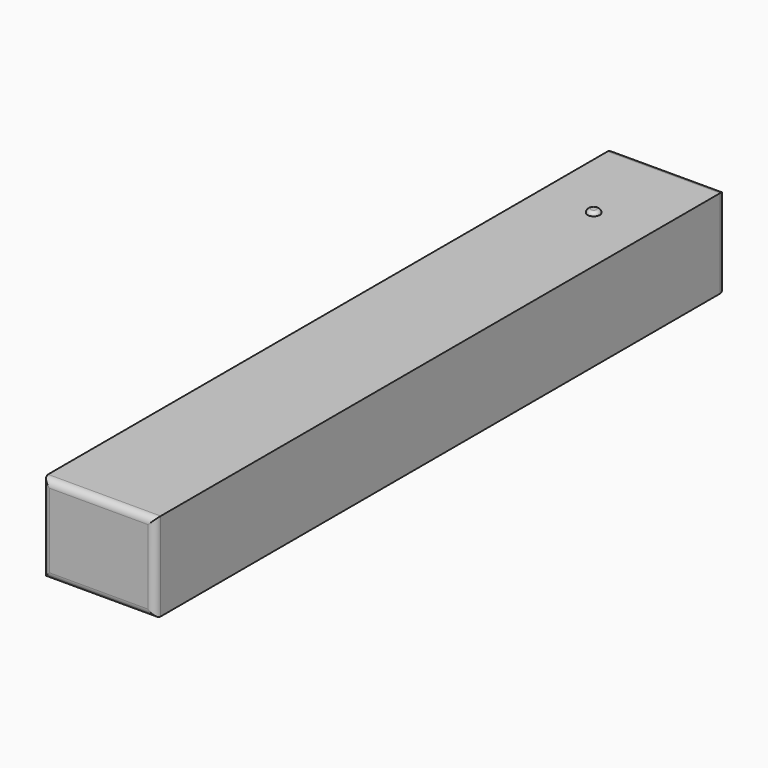
from build123d import *

# Parameters (mm, degrees)
F0_W      = 32.1
F0_H      = 25.2
F0_W_2    = 5.4
F0_H_2    = 5.4
F1_DEPTH  = 200
F3_W      = 32.1
F3_H      = 25.2
F4_DEPTH  = 3
F5_R      = 2
F6_R      = 1.75
F7_R      = 1.75
F8_DEPTH  = 1
F9_R      = 0.99999
F10_R     = 1.75
F11_DEPTH = 1
F12_R     = 0.99999


# Not quite as in the source:
# - a fillet or chamfer is up to 0.001 mm smaller than in the source, because OpenCascade refuses the exact size


with BuildPart() as f1:
    # F0 (on Front) → F1 (new body)
    with BuildSketch(Plane.XZ):
        with Locations((-0.710526225, -0.3999928176)):
            Rectangle(F0_W, F0_H)
        Polygon((-13.760526225, -6.9499006331), (-13.760526225, -4.5999928176), (-8.360526225, -4.5999928176), (-8.360526225, -9.9999928176), (-13.760526225, -9.9999928176), align=None, mode=Mode.SUBTRACT)
        with Locations((-4.160526225, -7.2999928176)):
            Rectangle(F0_W_2, F0_H_2, mode=Mode.SUBTRACT)
        Polygon((-13.760526225, -3.0999928176), (-13.760526225, 0.7499149978), (-13.760526225, 2.3000071824), (-8.360526225, 2.3000071824), (-8.360526225, -3.0999928176), align=None, mode=Mode.SUBTRACT)
        with Locations((-4.160526225, -0.3999928176)):
            Rectangle(F0_W_2, F0_H_2, mode=Mode.SUBTRACT)
        with Locations((2.739473775, -7.2999928176)):
            Rectangle(F0_W_2, F0_H_2, mode=Mode.SUBTRACT)
        with Locations((9.639473775, -7.2999928176)):
            Rectangle(F0_W_2, F0_H_2, mode=Mode.SUBTRACT)
        with Locations((2.739473775, -0.3999928176)):
            Rectangle(F0_W_2, F0_H_2, mode=Mode.SUBTRACT)
        with Locations((9.639473775, -0.3999928176)):
            Rectangle(F0_W_2, F0_H_2, mode=Mode.SUBTRACT)
        with Locations((-11.060526225, 6.5000071824)):
            Rectangle(F0_W_2, F0_H_2, mode=Mode.SUBTRACT)
        with Locations((-4.160526225, 6.5000071824)):
            Rectangle(F0_W_2, F0_H_2, mode=Mode.SUBTRACT)
        with Locations((2.739473775, 6.5000071824)):
            Rectangle(F0_W_2, F0_H_2, mode=Mode.SUBTRACT)
        with Locations((9.639473775, 6.5000071824)):
            Rectangle(F0_W_2, F0_H_2, mode=Mode.SUBTRACT)
    extrude(amount=F1_DEPTH)

    # F3 (on face) → F4 (join)
    with BuildSketch(Plane.XZ.offset(200)):
        with Locations((-0.710526225, -0.3999928176)):
            Rectangle(F3_W, F3_H)
    extrude(amount=F4_DEPTH)

    # F5
    f5_edges = [f1.edges().sort_by_distance(p)[0] for p in [
        (15.339474, -203, -0.399993),
        (-0.710526, -203, 12.200007),
        (-16.760526, -203, -0.399993),
        (-0.710526, -203, -12.999993),
    ]]
    fillet(f5_edges, radius=F5_R)

    # F6
    f6_edges = [f1.edges().sort_by_distance(p)[0] for p in [
        (-0.710526, 0, 12.200007),
        (15.339474, 0, -0.399993),
        (-0.710526, 0, -12.999993),
        (-16.760526, 0, -0.399993),
    ]]
    fillet(f6_edges, radius=F6_R)

    # F7 (on face) → F8 (join)
    with BuildSketch(Plane.XY.offset(12.2000071824)):
        with Locations((-0.710526225, -26.75)):
            Circle(F7_R)
    extrude(amount=F8_DEPTH)

    # F9 (radius 1 in the source; OpenCascade refuses exactly that, so slightly less here)
    f9_edges = [f1.edges().sort_by_distance(p)[0] for p in [
        (-2.460526, -26.75, 13.200007),
    ]]
    fillet(f9_edges, radius=F9_R)

    # F10 (on face) → F11 (join)
    with BuildSketch(Plane(origin=(0, 0, -12.9999928176), x_dir=(1, 0, 0), z_dir=(0, 0, -1))):
        with Locations((-0.710526225, 26.75)):
            Circle(F10_R)
    extrude(amount=F11_DEPTH)

    # F12 (radius 1 in the source; OpenCascade refuses exactly that, so slightly less here)
    f12_edges = [f1.edges().sort_by_distance(p)[0] for p in [
        (-2.460526, -26.75, -13.999993),
    ]]
    fillet(f12_edges, radius=F12_R)


solid = f1.part
